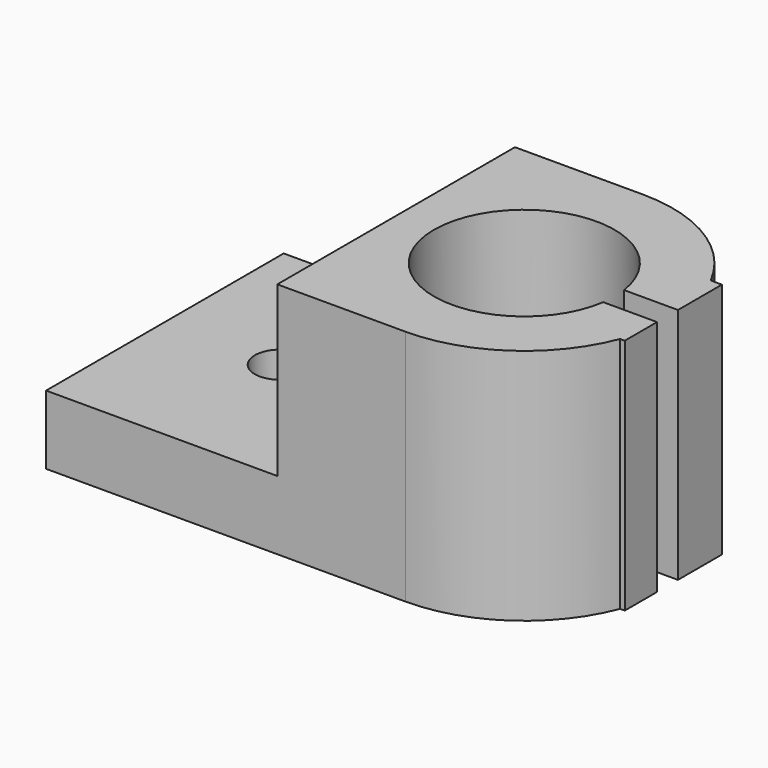
from build123d import *

# Parameters (mm, degrees)
F1_DEPTH = 20
F2_DEPTH = 5.8
F3_R     = 2.1592673483
F4_DEPTH = 25


# Not quite as in the source:
# - a feature names something its author has since deleted; it is built from what else it names


with BuildPart() as f1:
    # F0 (on Top) → F1 (new body)
    with BuildSketch(Plane.XY):
        with BuildLine():
            ThreePointArc((7.5199086274, -1.1004427451), (-7.6, 0), (7.5199086274, 1.1004427451))
            Line((7.5199086274, 1.1004427451), (12.0555223817, 1.1004427451))
            Line((12.0555223817, 1.1004427451), (12.0555223817, 5.7252630293))
            Line((12.0555223817, 5.7252630293), (11.1117668822, 5.7252630293))
            ThreePointArc((11.1117668822, 5.7252630293), (6.5070812248, 10.6727641187), (0, 12.5))
            Line((0, 12.5), (-10.78635397, 12.5))
            Line((-10.78635397, 12.5), (-10.78635397, 4.5))
            Line((-10.78635397, 4.5), (-10.78635397, -4.5))
            Line((-10.78635397, -4.5), (-10.78635397, -12.5))
            Line((-10.78635397, -12.5), (0, -12.5))
            ThreePointArc((0, -12.5), (7.0722638762, -10.3069434687), (11.6629478347, -4.4972933866))
            Line((11.6629478347, -4.4972933866), (12.0555223817, -4.4972933866))
            Line((12.0555223817, -4.4972933866), (12.0555223817, -1.1004427451))
            Line((12.0555223817, -1.1004427451), (7.5199086274, -1.1004427451))
        make_face()
    extrude(amount=F1_DEPTH)

    # F0 (on Top) → F2 (join)
    with BuildSketch(Plane.XY):
        Polygon((-10.78635397, 4.5), (-10.78635397, 12.5), (-30.2485086955, 12.5), (-30.2485086955, -4.5), (-30.2485086955, -12.5), (-10.78635397, -12.5), (-10.78635397, -4.5), align=None)
    extrude(amount=F2_DEPTH)

    # F3 (on face) → F4 (cut)
    with BuildSketch(Plane.XY.offset(5.8)):
        with Locations((-20.5174313327, 0)):
            Circle(F3_R)
    extrude(amount=-F4_DEPTH, mode=Mode.SUBTRACT)


solid = f1.part
